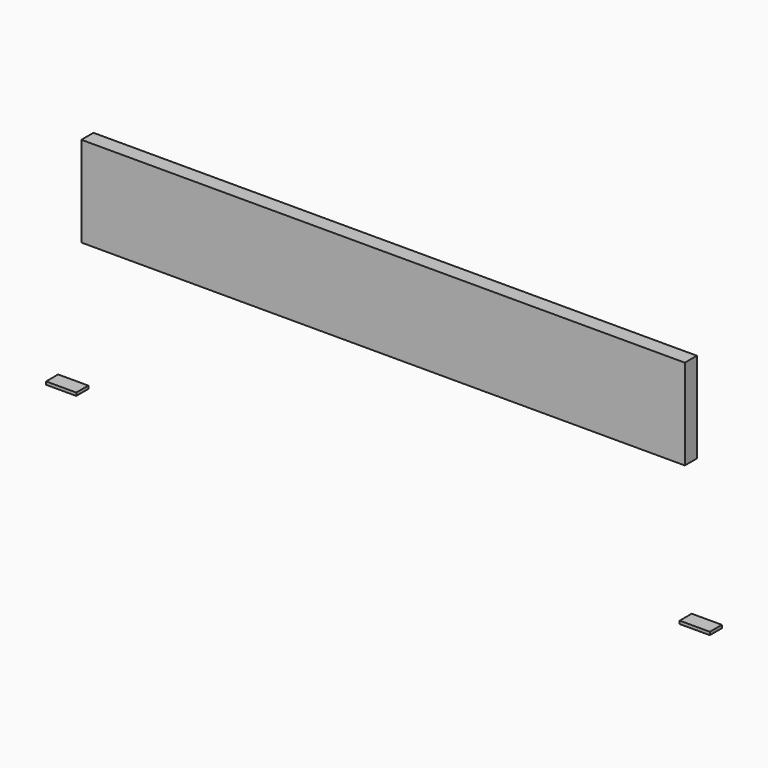
from build123d import *

# Parameters (mm, degrees)
F0_W     = 50
F0_H     = 5
F1_DEPTH = 25
F2_W     = 1000
F2_H     = 150
F3_DEPTH = 25


with BuildPart() as f1:
    # F0 (on Front) → F1 (new body)
    with BuildSketch(Plane.XZ):
        with Locations((-549.1185657559, -86.3759217312)):
            Rectangle(F0_W, F0_H)
    extrude(amount=F1_DEPTH)


with BuildPart() as f1b:
    # F0 (on Front) → F1, piece 2 (new body)
    with BuildSketch(Plane.XZ):
        with Locations((500.8814342441, -93.9516803368)):
            Rectangle(F0_W, F0_H)
    extrude(amount=F1_DEPTH)


with BuildPart() as f3:
    # F2 (on Front) → F3 (new body)
    with BuildSketch(Plane.XZ):
        with Locations((-15.6014859676, 212.6752244859)):
            Rectangle(F2_W, F2_H)
    extrude(amount=F3_DEPTH)


solid = Compound([f1.part, f1b.part, f3.part])
